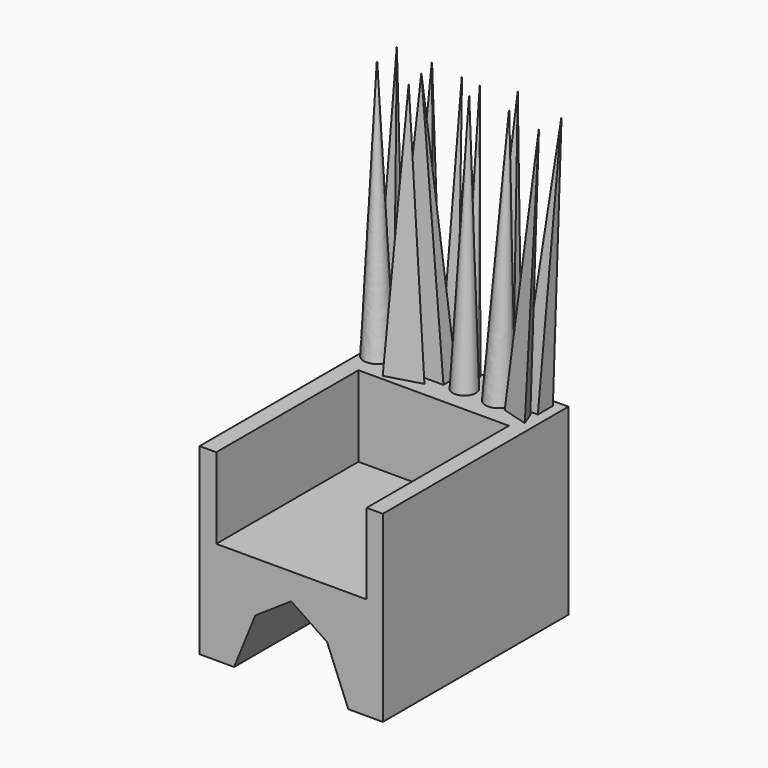
from build123d import *

# Parameters (mm, degrees)
F0_W         = 25
F0_H         = 25
F0_H_2       = 6.658737734
F1_DEPTH     = 25
F3_DEPTH     = 35.6
F4_W         = 2.6114728302
F4_H         = 1.8013045192
F4_W_2       = 7.1746204048
F4_H_2       = 2.2207163274
F4_W_3       = 3.8653127849
F4_H_3       = 1.3321898878
F4_R         = 1.5749223429
F4_R_2       = 1.7802160879
F4_W_4       = 2.5623645633
F4_H_4       = 2.5623627007
F20_DEPTH    = 11
F21_T1_DEPTH = 31.658737734


# Not quite as in the source:
# - a fillet or chamfer that OpenCascade refuses, or shapes differently, is made with other operations: its cross-section is extruded or revolved along the edge and cut away or added


with BuildPart() as f1:
    # F0 (on Top) → F1 (new body)
    with BuildSketch(Plane.XY):
        Rectangle(F0_W, F0_H)
        with Locations((0, 15.829368867)):
            Rectangle(F0_W, F0_H_2)
    extrude(amount=F1_DEPTH)

    # F2 (on face) → F3 (cut)
    with BuildSketch(Plane.XZ.offset(12.5)):
        Polygon((0, 11.7594422773), (0, 0), (7.7875177376, 0), (3.0218927836, 11.7594422773), align=None)
        Polygon((-3.0218927836, 11.7594422773), (-7.7875177376, 0), (0, 0), (0, 11.7594422773), align=None)
    extrude(amount=-F3_DEPTH, mode=Mode.SUBTRACT)

    # F4 (on face) → F7 section 0
    with BuildSketch(Plane.XY.offset(25), mode=Mode.PRIVATE) as f7_s0:
        with BuildLine():
            ThreePointArc((-8.8635824621, 15.5248958617), (-10.681791231, 17.3431046307), (-12.5, 15.5248958617))
            ThreePointArc((-12.5, 15.5248958617), (-10.681791231, 13.7066870928), (-8.8635824621, 15.5248958617))
        make_face()
    loft([f7_s0.sketch, Vertex(-11.7442617193, 16.8165676296, 60)])

    # F4 (on face) → F8 section 0
    with BuildSketch(Plane.XY.offset(25), mode=Mode.PRIVATE) as f8_s0:
        with Locations((-11.1942635849, 18.2580854744)):
            Rectangle(F4_W, F4_H)
    loft([f8_s0.sketch, Vertex(-11.7442617193, 20.1987158507, 60)])

    # F4 (on face) → F9 section 0
    with BuildSketch(Plane.XY.offset(25), mode=Mode.PRIVATE) as f9_s0:
        Polygon((11.2469336018, 13.2797770202), (10.5349393561, 15.1175186038), (7.6900690421, 14.3002654268), align=None)
    loft([Vertex(11.8099879473, 15.0047028437, 60), f9_s0.sketch])

    # F4 (on face) → F10 section 0
    with BuildSketch(Plane.XY.offset(25), mode=Mode.PRIVATE) as f10_s0:
        with Locations((-4.6175280586, 15.8665440977)):
            Rectangle(F4_W_2, F4_H_2)
    loft([f10_s0.sketch, Vertex(-5.8858972043, 17.0581489801, 60)])

    # F4 (on face) → F11 section 0
    with BuildSketch(Plane.XY.offset(25), mode=Mode.PRIVATE) as f11_s0:
        Polygon((-5.9617283097, 14.5839094924), (-7.3897121474, 12.3443854973), (-2.7514786925, 13.6628672481), align=None)
    loft([Vertex(-5.3423377685, 14.2195606604, 60), f11_s0.sketch])

    # F4 (on face) → F12 section 0
    with BuildSketch(Plane.XY.offset(25), mode=Mode.PRIVATE) as f12_s0:
        with Locations((-6.4965952188, 18.1957688183)):
            Rectangle(F4_W_3, F4_H_3)
    loft([f12_s0.sketch, Vertex(-6.8522254005, 20.0779251754, 60)])

    # F4 (on face) → F13 section 0
    with BuildSketch(Plane.XY.offset(25), mode=Mode.PRIVATE) as f13_s0:
        Polygon((-1.36240758, 17.6026448607), (-2.6916782372, 19.158737734), (-3.5105766729, 17.2970890999), align=None)
    loft([f13_s0.sketch, Vertex(-2.5037485175, 19.7759475559, 60)])

    # F4 (on face) → F14 section 0
    with BuildSketch(Plane.XY.offset(25), mode=Mode.PRIVATE) as f14_s0:
        with Locations((1.2759102974, 15.4394833371)):
            Circle(F4_R)
    loft([Vertex(1.1199823348, 16.4541937411, 60), f14_s0.sketch])

    # F4 (on face) → F15 section 0
    with BuildSketch(Plane.XY.offset(25), mode=Mode.PRIVATE) as f15_s0:
        with BuildLine():
            ThreePointArc((0.9860657156, 18.1726720184), (0.6972537523, 18.8699257744), (-5.2e-09, 19.158737734))
            ThreePointArc((-5.2e-09, 19.158737734), (-0.6972537523, 17.4754182624), (0.9860657156, 18.1726720184))
        make_face()
    loft([Vertex(-0.0879280269, 19.8363438249, 60), f15_s0.sketch])

    # F4 (on face) → F16 section 0
    with BuildSketch(Plane.XY.offset(25), mode=Mode.PRIVATE) as f16_s0:
        Polygon((6.14440348, 19.158737734), (2.386267297, 19.158737734), (2.386267297, 17.3574332148), (6.14440348, 17.6535397768), align=None)
    loft([Vertex(4.8041078262, 20.1383195817, 60), f16_s0.sketch])

    # F4 (on face) → F17 section 0
    with BuildSketch(Plane.XY.offset(25), mode=Mode.PRIVATE) as f17_s0:
        with Locations((5.8027543128, 15.6103083864)):
            Circle(F4_R_2)
    loft([Vertex(6.4347875305, 16.6353806853, 60), f17_s0.sketch])

    # F4 (on face) → F18 section 0
    with BuildSketch(Plane.XY.offset(25), mode=Mode.PRIVATE) as f18_s0:
        with Locations((9.8171252757, 16.9769022614)):
            Rectangle(F4_W_4, F4_H_4)
    loft([f18_s0.sketch, Vertex(11.9911748916, 18.6284333467, 60)])

    # F19 (on face) → F20 (cut)
    with BuildSketch(Plane.XY.offset(25)):
        Polygon((10.2956090122, -14.3586313352), (10.2956090122, -12.4287493527), (10.2956090122, 11.7455618456), (-10.2220848203, 11.7455618456), (-10.2220848203, -12.3271765187), (-10.2220848203, -14.3586313352), align=None)
    extrude(amount=-F20_DEPTH, mode=Mode.SUBTRACT)

    # F21: chamfer of 5 on 2 edges, made by hand

    # F21_s2 → F21_t1 (join)
    with BuildSketch(Plane.XZ.offset(-19.158737734)):
        Polygon((-4.8998373819, 7.1255104601), (1.9781072164, 11.7594422773), (-3.0218927836, 11.7594422773), align=None)
        Polygon((-1.9781072164, 11.7594422773), (4.8998373819, 7.1255104601), (3.0218927836, 11.7594422773), align=None)
    extrude(amount=F21_T1_DEPTH)


solid = f1.part
